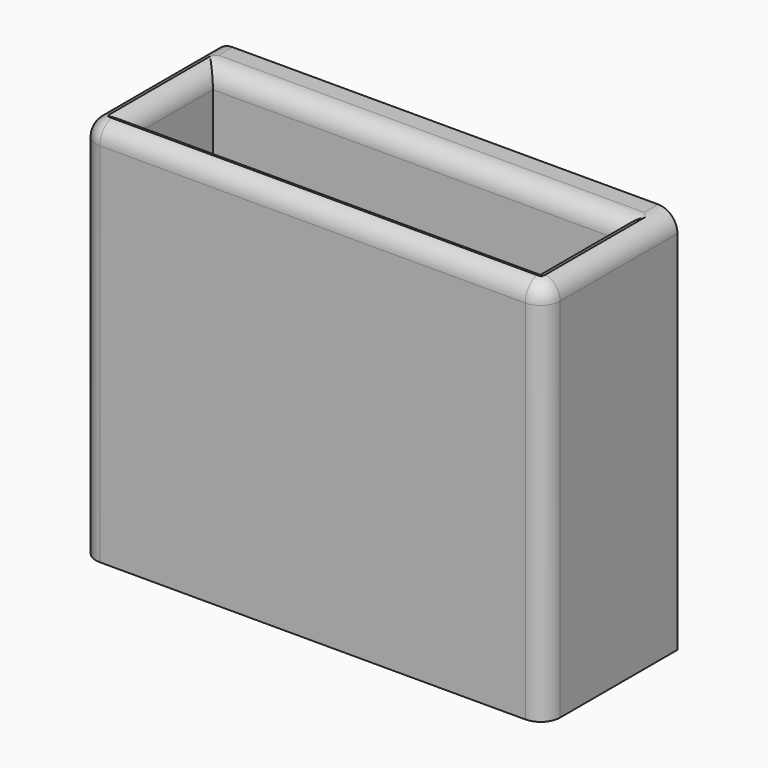
from build123d import *

# Parameters (mm, degrees)
F1_DEPTH      = 6.4
F2_R          = 6.4
F3_DEPTH      = 0.5
F5_DEPTH      = 35
F5_DEPTH_BACK = 5
F6_T          = -3
F7_W          = 48.1
F7_H          = 40
F8_DEPTH      = 10
F9_T1_DEPTH   = 22.4
F9_T3_DEPTH   = 44.1
F9_T5_DEPTH   = 10.4
F9_T7_DEPTH   = 42.1
F9_T9_DEPTH   = 43
F9_S13_W      = 2
F9_S13_H      = 2
F9_T14_DEPTH  = 2
F9_S19_W      = 2
F9_S19_H      = 2
F9_T20_DEPTH  = 2
F9_S25_W      = 2
F9_S25_H      = 2
F9_T26_DEPTH  = 2
F9_S31_W      = 2
F9_S31_H      = 2
F9_T32_DEPTH  = 2
F9_T39_DEPTH  = 15.4
F9_T43_DEPTH  = 47.1
F9_T50_DEPTH  = 15.4
F9_T54_DEPTH  = 47.1
F9_T61_DEPTH  = 47.1
F9_T65_DEPTH  = 15.4
F9_T72_DEPTH  = 15.4
F9_T76_DEPTH  = 47.1
F11_W         = 65.6272098422
F11_H         = 14.6678336896
F12_DEPTH     = 40.001


# Not quite as in the source:
# - a fillet or chamfer that OpenCascade refuses, or shapes differently, is made with other operations: its cross-section is extruded or revolved along the edge and cut away or added


with BuildPart() as f1:
    # F0 (on Front) → F1 (new body)
    with BuildSketch(Plane.XZ):
        with BuildLine():
            ThreePointArc((19.05, 57.1), (17.5855339059, 60.6355339059), (14.05, 62.1))
            Line((14.05, 62.1), (-14.05, 62.1))
            ThreePointArc((-14.05, 62.1), (-17.5855339059, 60.6355339059), (-19.05, 57.1))
            Line((-19.05, 57.1), (-19.05, -57.1))
            ThreePointArc((-19.05, -57.1), (-17.5855339059, -60.6355339059), (-14.05, -62.1))
            Line((-14.05, -62.1), (14.05, -62.1))
            ThreePointArc((14.05, -62.1), (17.5855339059, -60.6355339059), (19.05, -57.1))
            Line((19.05, -57.1), (19.05, 57.1))
        make_face()
    extrude(amount=F1_DEPTH)

    # F2 (on face) → F3 (join)
    with BuildSketch(Plane.XZ.offset(6.4)):
        with BuildLine():
            ThreePointArc((1.6, 0), (8, -6.4), (14.4, 0))
            ThreePointArc((14.4, 0), (8, 6.4), (1.6, 0))
        make_face()
        with BuildLine():
            Line((14.4, -16.1), (14.4, 0))
            ThreePointArc((14.4, 0), (8, -6.4), (1.6, 0))
            Line((1.6, 0), (1.6, -16.1))
            ThreePointArc((1.6, -16.1), (8, -9.7), (14.4, -16.1))
        make_face()
        with BuildLine():
            ThreePointArc((1.6, -16.1), (8, -22.5), (14.4, -16.1))
            ThreePointArc((14.4, -16.1), (8, -9.7), (1.6, -16.1))
        make_face()
        with Locations((8, 16.1)):
            Circle(F2_R)
        with Locations((-8, 16.1)):
            Circle(F2_R)
        with Locations((-8, 0)):
            Circle(F2_R)
        with Locations((-8, -16.1)):
            Circle(F2_R)
    extrude(amount=F3_DEPTH)


with BuildPart() as f5:
    # F4 (on face) → F5 (new body, two sides)
    with BuildSketch(Plane(origin=(0, 0, -62.1), x_dir=(1, 0, 0), z_dir=(0, 0, -1))) as f5_sk:
        Polygon((-14.05, 11.4), (-24.05, 11.4), (-24.05, -5), (-14.05, -5), (14.05, -5), (24.05, -5), (24.05, 11.4), (14.05, 11.4), align=None)
    extrude(amount=-F5_DEPTH)
    extrude(f5_sk.sketch, amount=F5_DEPTH_BACK)

    # F6
    f6_openings = [f5.faces().sort_by_distance(p)[0] for p in [
        (0, -3.2, -27.1),
    ]]
    offset(amount=F6_T, openings=f6_openings)

    # F7 (on face) → F8 (join)
    with BuildSketch(Plane(origin=(0, 5, 0), x_dir=(-1, 0, 0), z_dir=(0, 1, 0))):
        with Locations((0, -47.1)):
            Rectangle(F7_W, F7_H)
    extrude(amount=F8_DEPTH)

    # F9: fillet of radius 2 on 12 edges, made by hand

    # F9_s2 → F9_t1 (cut)
    with BuildSketch(Plane.XZ.offset(-13)):
        with BuildLine():
            ThreePointArc((-24.05, -29.1), (-23.4642135624, -27.6857864376), (-22.05, -27.1))
            Line((-22.05, -27.1), (-24.05, -27.1))
            Line((-24.05, -27.1), (-24.05, -29.1))
        make_face()
        with BuildLine():
            ThreePointArc((24.05, -29.1), (23.4642135624, -27.6857864376), (22.05, -27.1))
            Line((22.05, -27.1), (24.05, -27.1))
            Line((24.05, -27.1), (24.05, -29.1))
        make_face()
    extrude(amount=F9_T1_DEPTH, mode=Mode.SUBTRACT)

    # F9_s4 → F9_t3 (cut)
    with BuildSketch(Plane.YZ.offset(-22.05)):
        with BuildLine():
            ThreePointArc((15, -29.1), (14.4142135624, -27.6857864376), (13, -27.1))
            Line((13, -27.1), (15, -27.1))
            Line((15, -27.1), (15, -29.1))
        make_face()
        with BuildLine():
            ThreePointArc((-11.4, -29.1), (-10.8142135624, -27.6857864376), (-9.4, -27.1))
            Line((-9.4, -27.1), (-11.4, -27.1))
            Line((-11.4, -27.1), (-11.4, -29.1))
        make_face()
    extrude(amount=F9_T3_DEPTH, mode=Mode.SUBTRACT)

    # F9_s6 → F9_t5 (cut)
    with BuildSketch(Plane.XZ.offset(-2)):
        with BuildLine():
            ThreePointArc((-23.05, -27.1), (-21.6357864376, -27.6857864376), (-21.05, -29.1))
            Line((-21.05, -29.1), (-21.05, -27.1))
            Line((-21.05, -27.1), (-23.05, -27.1))
        make_face()
        with BuildLine():
            ThreePointArc((23.05, -27.1), (21.6357864376, -27.6857864376), (21.05, -29.1))
            Line((21.05, -29.1), (21.05, -27.1))
            Line((21.05, -27.1), (23.05, -27.1))
        make_face()
    extrude(amount=F9_T5_DEPTH, mode=Mode.SUBTRACT)

    # F9_s8 → F9_t7 (cut)
    with BuildSketch(Plane.YZ.offset(-21.05)):
        with BuildLine():
            ThreePointArc((-10.4, -27.1), (-8.9857864376, -27.6857864376), (-8.4, -29.1))
            Line((-8.4, -29.1), (-8.4, -27.1))
            Line((-8.4, -27.1), (-10.4, -27.1))
        make_face()
        with BuildLine():
            ThreePointArc((4, -27.1), (2.5857864376, -27.6857864376), (2, -29.1))
            Line((2, -29.1), (2, -27.1))
            Line((2, -27.1), (4, -27.1))
        make_face()
    extrude(amount=F9_T7_DEPTH, mode=Mode.SUBTRACT)

    # F9_s10 → F9_t9 (cut)
    with BuildSketch(Plane.XY.offset(-72.1)):
        with BuildLine():
            ThreePointArc((22.05, -11.4), (23.4642135624, -10.8142135624), (24.05, -9.4))
            Line((24.05, -9.4), (24.05, -11.4))
            Line((24.05, -11.4), (22.05, -11.4))
        make_face()
        with BuildLine():
            ThreePointArc((24.05, 13), (23.4642135624, 14.4142135624), (22.05, 15))
            Line((22.05, 15), (24.05, 15))
            Line((24.05, 15), (24.05, 13))
        make_face()
        with BuildLine():
            ThreePointArc((-22.05, 15), (-23.4642135624, 14.4142135624), (-24.05, 13))
            Line((-24.05, 13), (-24.05, 15))
            Line((-24.05, 15), (-22.05, 15))
        make_face()
        with BuildLine():
            ThreePointArc((-22.05, -11.4), (-23.4642135624, -10.8142135624), (-24.05, -9.4))
            Line((-24.05, -9.4), (-24.05, -11.4))
            Line((-24.05, -11.4), (-22.05, -11.4))
        make_face()
    extrude(amount=F9_T9_DEPTH, mode=Mode.SUBTRACT)


with BuildPart() as f9_tool12:
    # F9_s13 → F9_t14 (new body)
    with BuildSketch(Plane.XZ.offset(-13)):
        with Locations((-23.05, -28.1)):
            Rectangle(F9_S13_W, F9_S13_H)
    extrude(amount=-F9_T14_DEPTH)

    # F9_s15 → F9_t16 (revolve, cut)
    with BuildSketch(Plane(origin=(-22.05, 13, -29.1), x_dir=(0.7071067812, 0, -0.7071067812), z_dir=(0.7071067812, 0, 0.7071067812))):
        with BuildLine():
            ThreePointArc((0, -2), (2, 0), (0, 2))
            Line((0, 2), (0, -2))
        make_face()
    revolve(axis=Axis((-22.05, 13, -29.1), (0, 1, 0)), mode=Mode.SUBTRACT)


with BuildPart() as f5_1:
    add(f5.part)

    # F9_t11: cut F9_tool12
    add(f9_tool12.part, mode=Mode.SUBTRACT)


with BuildPart() as f9_tool18:
    # F9_s19 → F9_t20 (new body)
    with BuildSketch(Plane.XZ.offset(9.4)):
        with Locations((-23.05, -28.1)):
            Rectangle(F9_S19_W, F9_S19_H)
    extrude(amount=F9_T20_DEPTH)

    # F9_s21 → F9_t22 (revolve, cut)
    with BuildSketch(Plane(origin=(-22.05, -9.4, -29.1), x_dir=(0.7071067812, 0, -0.7071067812), z_dir=(-0.7071067812, 0, -0.7071067812))):
        with BuildLine():
            ThreePointArc((0, -2), (2, 0), (0, 2))
            Line((0, 2), (0, -2))
        make_face()
    revolve(axis=Axis((-22.05, -9.4, -29.1), (0, -1, 0)), mode=Mode.SUBTRACT)


with BuildPart() as f5_2:
    add(f5_1.part)

    # F9_t17: cut F9_tool18
    add(f9_tool18.part, mode=Mode.SUBTRACT)


with BuildPart() as f9_tool24:
    # F9_s25 → F9_t26 (new body)
    with BuildSketch(Plane.YZ.offset(22.05)):
        with Locations((14, -28.1)):
            Rectangle(F9_S25_W, F9_S25_H)
    extrude(amount=F9_T26_DEPTH)

    # F9_s27 → F9_t28 (revolve, cut)
    with BuildSketch(Plane(origin=(22.05, 13, -29.1), x_dir=(0, -0.7071067812, -0.7071067812), z_dir=(0, -0.7071067812, 0.7071067812))):
        with BuildLine():
            ThreePointArc((0, -2), (2, 0), (0, 2))
            Line((0, 2), (0, -2))
        make_face()
    revolve(axis=Axis((22.05, 13, -29.1), (1, 0, 0)), mode=Mode.SUBTRACT)


with BuildPart() as f5_3:
    add(f5_2.part)

    # F9_t23: cut F9_tool24
    add(f9_tool24.part, mode=Mode.SUBTRACT)


with BuildPart() as f9_tool30:
    # F9_s31 → F9_t32 (new body)
    with BuildSketch(Plane.XZ.offset(9.4)):
        with Locations((23.05, -28.1)):
            Rectangle(F9_S31_W, F9_S31_H)
    extrude(amount=F9_T32_DEPTH)

    # F9_s33 → F9_t34 (revolve, cut)
    with BuildSketch(Plane(origin=(22.05, -9.4, -29.1), x_dir=(-0.7071067812, 0, -0.7071067812), z_dir=(-0.7071067812, 0, 0.7071067812))):
        with BuildLine():
            ThreePointArc((0, -2), (2, 0), (0, 2))
            Line((0, 2), (0, -2))
        make_face()
    revolve(axis=Axis((22.05, -9.4, -29.1), (0, -1, 0)), mode=Mode.SUBTRACT)


with BuildPart() as f5_4:
    add(f5_3.part)

    # F9_t29: cut F9_tool30
    add(f9_tool30.part, mode=Mode.SUBTRACT)


with BuildPart() as f9_tool37:
    # F9_s38 → F9_t39 (new body)
    with BuildSketch(Plane.XZ.offset(13.4)):
        with BuildLine():
            ThreePointArc((-23.05, -27.1), (-21.6357864376, -27.6857864376), (-21.05, -29.1))
            Line((-21.05, -29.1), (-21.05, -27.1))
            Line((-21.05, -27.1), (-23.05, -27.1))
        make_face()
    extrude(amount=-F9_T39_DEPTH)

    split(bisect_by=Plane.XZ.offset(8.4), keep=Keep.TOP)


with BuildPart() as f9_tool41:
    # F9_s42 → F9_t43 (new body)
    with BuildSketch(Plane.YZ.offset(21.05)):
        with BuildLine():
            ThreePointArc((-10.4, -27.1), (-8.9857864376, -27.6857864376), (-8.4, -29.1))
            Line((-8.4, -29.1), (-8.4, -27.1))
            Line((-8.4, -27.1), (-10.4, -27.1))
        make_face()
    extrude(amount=-F9_T43_DEPTH)

    split(bisect_by=Plane.YZ.offset(-21.05), keep=Keep.BOTTOM)


with BuildPart() as f9_tool37_1:
    add(f9_tool37.part)

    # F9_t45: intersect F9_tool41
    add(f9_tool41.part, mode=Mode.INTERSECT)


with BuildPart() as f5_5:
    add(f5_4.part)

    # F9_t35: cut F9_tool37
    add(f9_tool37_1.part, mode=Mode.SUBTRACT)


with BuildPart() as f9_tool48:
    # F9_s49 → F9_t50 (new body)
    with BuildSketch(Plane.XZ.offset(8.4)):
        with BuildLine():
            ThreePointArc((-23.05, -27.1), (-21.6357864376, -27.6857864376), (-21.05, -29.1))
            Line((-21.05, -29.1), (-21.05, -27.1))
            Line((-21.05, -27.1), (-23.05, -27.1))
        make_face()
    extrude(amount=-F9_T50_DEPTH)

    split(bisect_by=Plane.XZ.offset(-2), keep=Keep.BOTTOM)


with BuildPart() as f9_tool52:
    # F9_s53 → F9_t54 (new body)
    with BuildSketch(Plane.YZ.offset(-26.05)):
        with BuildLine():
            ThreePointArc((4, -27.1), (2.5857864376, -27.6857864376), (2, -29.1))
            Line((2, -29.1), (2, -27.1))
            Line((2, -27.1), (4, -27.1))
        make_face()
    extrude(amount=F9_T54_DEPTH)

    split(bisect_by=Plane.YZ.offset(-21.05), keep=Keep.BOTTOM)


with BuildPart() as f9_tool48_1:
    add(f9_tool48.part)

    # F9_t56: intersect F9_tool52
    add(f9_tool52.part, mode=Mode.INTERSECT)


with BuildPart() as f5_6:
    add(f5_5.part)

    # F9_t46: cut F9_tool48
    add(f9_tool48_1.part, mode=Mode.SUBTRACT)


with BuildPart() as f9_tool59:
    # F9_s60 → F9_t61 (new body)
    with BuildSketch(Plane.YZ.offset(26.05)):
        with BuildLine():
            ThreePointArc((-10.4, -27.1), (-8.9857864376, -27.6857864376), (-8.4, -29.1))
            Line((-8.4, -29.1), (-8.4, -27.1))
            Line((-8.4, -27.1), (-10.4, -27.1))
        make_face()
    extrude(amount=-F9_T61_DEPTH)

    split(bisect_by=Plane.YZ.offset(21.05), keep=Keep.TOP)


with BuildPart() as f9_tool63:
    # F9_s64 → F9_t65 (new body)
    with BuildSketch(Plane.XZ.offset(-2)):
        with BuildLine():
            ThreePointArc((23.05, -27.1), (21.6357864376, -27.6857864376), (21.05, -29.1))
            Line((21.05, -29.1), (21.05, -27.1))
            Line((21.05, -27.1), (23.05, -27.1))
        make_face()
    extrude(amount=F9_T65_DEPTH)

    split(bisect_by=Plane.XZ.offset(8.4), keep=Keep.TOP)


with BuildPart() as f9_tool59_1:
    add(f9_tool59.part)

    # F9_t67: intersect F9_tool63
    add(f9_tool63.part, mode=Mode.INTERSECT)


with BuildPart() as f5_7:
    add(f5_6.part)

    # F9_t57: cut F9_tool59
    add(f9_tool59_1.part, mode=Mode.SUBTRACT)


with BuildPart() as f9_tool70:
    # F9_s71 → F9_t72 (new body)
    with BuildSketch(Plane.XZ.offset(-7)):
        with BuildLine():
            ThreePointArc((23.05, -27.1), (21.6357864376, -27.6857864376), (21.05, -29.1))
            Line((21.05, -29.1), (21.05, -27.1))
            Line((21.05, -27.1), (23.05, -27.1))
        make_face()
    extrude(amount=F9_T72_DEPTH)

    split(bisect_by=Plane.XZ.offset(-2), keep=Keep.BOTTOM)


with BuildPart() as f9_tool74:
    # F9_s75 → F9_t76 (new body)
    with BuildSketch(Plane.YZ.offset(-21.05)):
        with BuildLine():
            ThreePointArc((4, -27.1), (2.5857864376, -27.6857864376), (2, -29.1))
            Line((2, -29.1), (2, -27.1))
            Line((2, -27.1), (4, -27.1))
        make_face()
    extrude(amount=F9_T76_DEPTH)

    split(bisect_by=Plane.YZ.offset(21.05), keep=Keep.TOP)


with BuildPart() as f9_tool70_1:
    add(f9_tool70.part)

    # F9_t78: intersect F9_tool74
    add(f9_tool74.part, mode=Mode.INTERSECT)


with BuildPart() as f5_8:
    add(f5_7.part)

    # F9_t68: cut F9_tool70
    add(f9_tool70_1.part, mode=Mode.SUBTRACT)

    # F11 (on face) → F12 (cut, through all)
    with BuildSketch(Plane.XY.offset(-27.1)):
        with Locations((-0.3663264215, 13.1452779751)):
            Rectangle(F11_W, F11_H)
    extrude(amount=-F12_DEPTH, mode=Mode.SUBTRACT)


solid = f5_8.part
